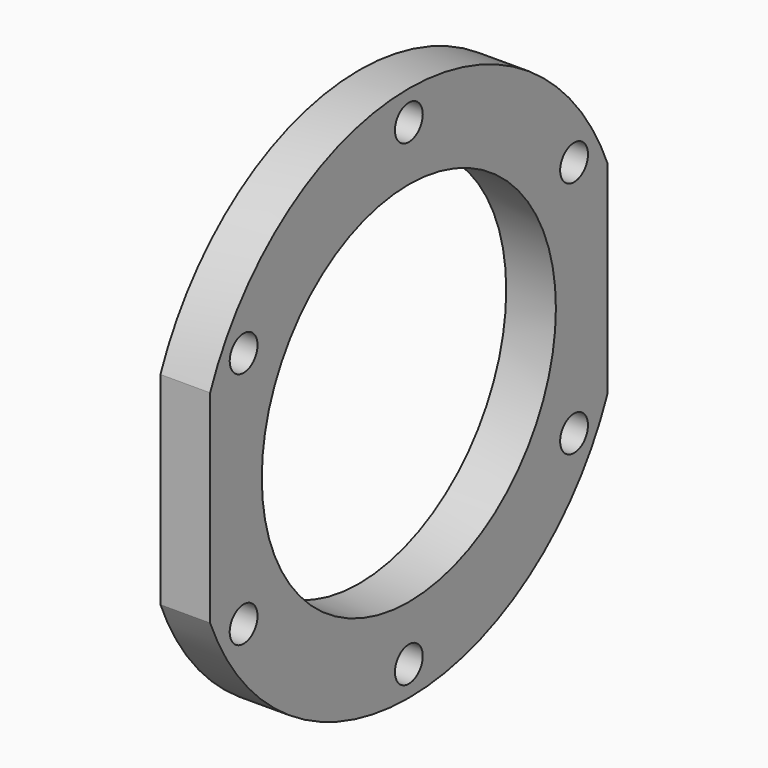
from build123d import *

# Parameters (mm, degrees)
F0_W            = 10
F0_H            = 17
F2_R            = 3.5
F3_DEPTH        = 10.001
F3_COPIES_COUNT = 6
F5_DEPTH        = 10.001


# Not quite as in the source:
# - a pattern or mirror of a feature is missing from the dataset's text; its kind, count and spacing are read off the source's solid


with BuildPart() as f1:
    # F0 (on Front) → F1 (revolve)
    with BuildSketch(Plane.XZ):
        with Locations((5, 45.5)):
            Rectangle(F0_W, F0_H)
    revolve(axis=Axis((-28.7704151153, 0, 0), (-1, 0, 0)))

    # F2 (on face) → F3 (cut, through all)
    with BuildSketch(Plane(origin=(0, 0, 0), x_dir=(0, -1, 0), z_dir=(-1, 0, 0))):
        with Locations((41.5692193817, 24)):
            Circle(F2_R)
    f3 = extrude(amount=-F3_DEPTH, mode=Mode.SUBTRACT)

    # F3_copies: F3 ×6 about axis
    f3_copies_axis = Axis((0, 0, 0), (1, 0, 0))
    for i in range(1, F3_COPIES_COUNT):
        add(f3.rotate(f3_copies_axis, i * 360 / F3_COPIES_COUNT), mode=Mode.SUBTRACT)

    # F4 (on face) → F5 (cut, through all)
    with BuildSketch(Plane(origin=(0, 0, 0), x_dir=(0, -1, 0), z_dir=(-1, 0, 0))):
        with BuildLine():
            Line((-50, -20.3960780544), (-50, 20.3960780544))
            ThreePointArc((-50, 20.3960780544), (-54, 0), (-50, -20.3960780544))
        make_face()
        with BuildLine():
            ThreePointArc((54, 0), (52.990565198, 10.3923048454), (50, 20.3960780544))
            Line((50, 20.3960780544), (50, -20.3960780544))
            ThreePointArc((50, -20.3960780544), (52.990565198, -10.3923048454), (54, 0))
        make_face()
    extrude(amount=-F5_DEPTH, mode=Mode.SUBTRACT)


solid = f1.part
